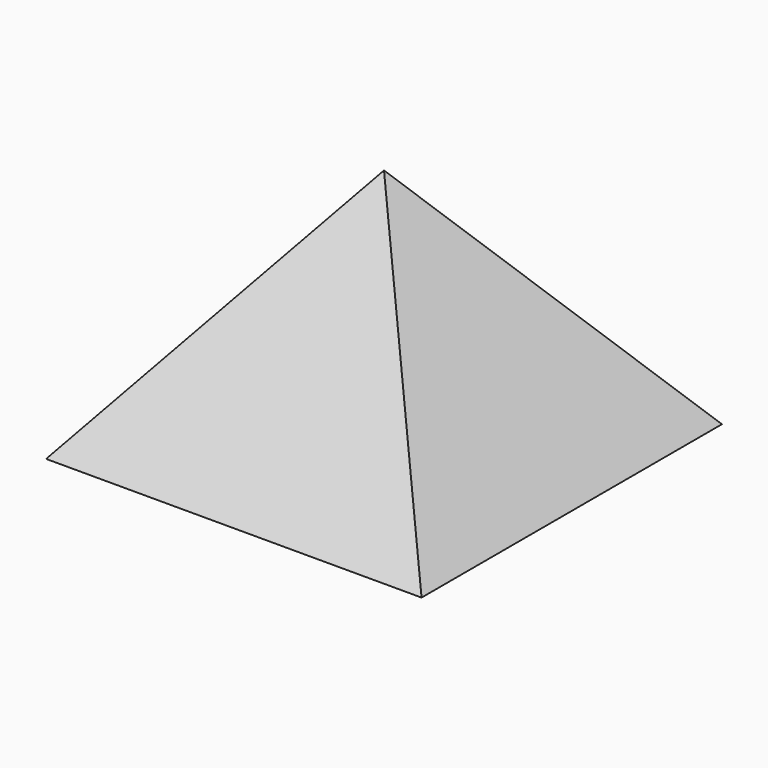
from build123d import *

# Parameters (mm, degrees)
F0_W     = 230398.32
F0_H     = 230398.32
F1_DEPTH = 146486.88
F2_SIZE2 = 146486.87999
F2_SIZE  = 115199.15999


# Not quite as in the source:
# - a fillet or chamfer is up to 0.001 mm smaller than in the source, because OpenCascade refuses the exact size


with BuildPart() as f1:
    # F0 (on Top) → F1 (new body)
    with BuildSketch(Plane.XY):
        Rectangle(F0_W, F0_H)
    extrude(amount=F1_DEPTH)

    # F2 (size 115199.16 and 146486.88 in the source; OpenCascade refuses exactly that, so slightly less here)
    f2_edges = [f1.edges().sort_by_distance(p)[0] for p in [
        (115199.16, 0, 146486.88),
        (0, 115199.16, 146486.88),
        (-115199.16, 0, 146486.88),
        (0, -115199.16, 146486.88),
    ]]
    f2_side = f1.faces().sort_by_distance((0, 0, 146486.88))[0]
    chamfer(f2_edges, length=F2_SIZE, length2=F2_SIZE2, reference=f2_side)


solid = f1.part
